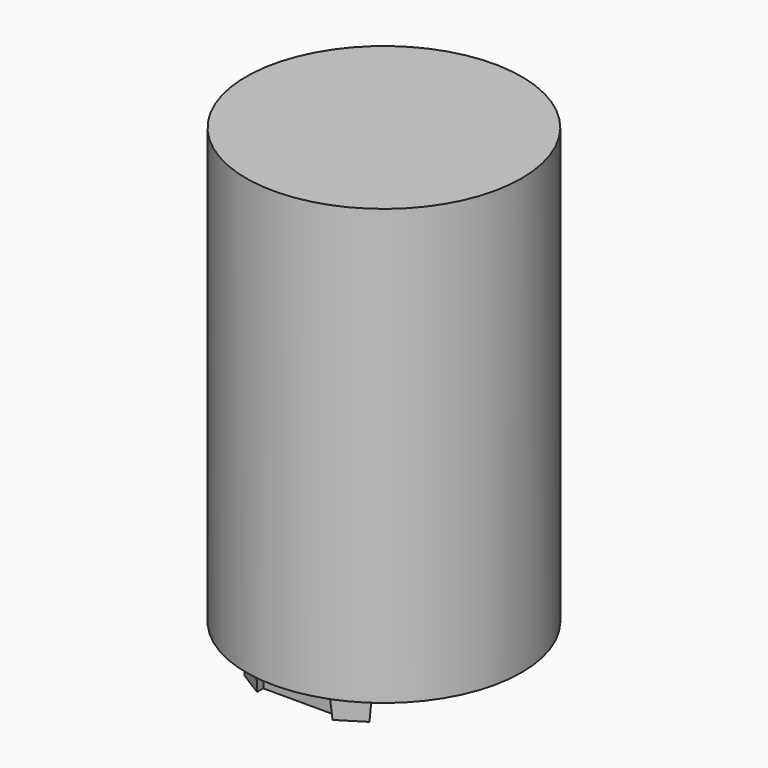
from build123d import *

# Parameters (mm, degrees)
F1_DEPTH = 2
F1_TAPER = 3
F0_R     = 9.5
F2_DEPTH = 30


with BuildPart() as f1:
    # F0 (on Top) → F1 (new body)
    with BuildSketch(Plane.XY):
        with BuildLine():
            Line((-2.5, -4.5), (-1.25, -4.5))
            Line((-1.25, -4.5), (-1.25, 8))
            ThreePointArc((-1.25, 8), (-1.6246096615, 8.4544378581), (-2.1421771094, 8.1734216623))
            Line((-2.1421771094, 8.1734216623), (-7.2625718321, -4.5))
            Line((-7.2625718321, -4.5), (-6.0125718321, -4.5))
            Line((-6.0125718321, -4.5), (-5.0025062675, -2))
            Line((-5.0025062675, -2), (-2.5, -2))
            Line((-2.5, -2), (-2.5, -4.5))
        make_face()
        Polygon((-2.5, -0.75), (-4.4974734852, -0.75), (-2.5, 4.1939203632), align=None, mode=Mode.SUBTRACT)
    extrude(amount=-F1_DEPTH, taper=F1_TAPER)


with BuildPart() as f1b:
    # F0 (on Top) → F1, piece 2 (new body)
    with BuildSketch(Plane.XY):
        with BuildLine():
            Line((1.25, 8.4544378581), (1.25, -4.5))
            ThreePointArc((1.25, -4.5), (5.075982109, -2.1148576985), (6.75, 2.0713944437))
            ThreePointArc((6.75, 2.0713944437), (5.1224940234, 6.2301220319), (1.25, 8.4544378581))
        make_face()
        with BuildLine():
            ThreePointArc((2.5, 6.7258275142), (4.6257418552, 4.8128070407), (5.4982695285, 2.0893678132))
            ThreePointArc((5.4982695285, 2.0893678132), (4.5914102703, -0.6620430511), (2.5, -2.6667022589))
            Line((2.5, -2.6667022589), (2.5, 6.7258275142))
        make_face(mode=Mode.SUBTRACT)
    extrude(amount=-F1_DEPTH, taper=F1_TAPER)


with BuildPart() as f1c:
    # F0 (on Top) → F1, piece 3 (new body)
    with BuildSketch(Plane.XY):
        Polygon((2.5, -6), (-2.5, -6), (-2.5, -5.375), (-4.5, -6.625), (-2.5, -7.875), (-2.5, -7.25), (2.5, -7.25), (2.5, -7.875), (4.5, -6.625), (2.5, -5.375), align=None)
    extrude(amount=-F1_DEPTH, taper=F1_TAPER)


with BuildPart() as f2:
    # F0 (on Top) → F2 (new body)
    with BuildSketch(Plane.XY):
        Circle(F0_R)
        Polygon((-2.5, -5.375), (-2.5, -6), (2.5, -6), (2.5, -5.375), (4.5, -6.625), (2.5, -7.875), (2.5, -7.25), (-2.5, -7.25), (-2.5, -7.875), (-4.5, -6.625), align=None, mode=Mode.SUBTRACT)
        with BuildLine():
            Line((-1.25, 8), (-1.25, -4.5))
            Line((-1.25, -4.5), (-2.5, -4.5))
            Line((-2.5, -4.5), (-2.5, -2))
            Line((-2.5, -2), (-5.0025062675, -2))
            Line((-5.0025062675, -2), (-6.0125718321, -4.5))
            Line((-6.0125718321, -4.5), (-7.2625718321, -4.5))
            Line((-7.2625718321, -4.5), (-2.1421771094, 8.1734216623))
            ThreePointArc((-2.1421771094, 8.1734216623), (-1.6246096615, 8.4544378581), (-1.25, 8))
        make_face(mode=Mode.SUBTRACT)
        with BuildLine():
            ThreePointArc((6.75, 2.0713944437), (5.075982109, -2.1148576985), (1.25, -4.5))
            Line((1.25, -4.5), (1.25, 8.4544378581))
            ThreePointArc((1.25, 8.4544378581), (5.1224940234, 6.2301220319), (6.75, 2.0713944437))
        make_face(mode=Mode.SUBTRACT)
        with BuildLine():
            Line((1.25, 8.4544378581), (1.25, -4.5))
            ThreePointArc((1.25, -4.5), (5.075982109, -2.1148576985), (6.75, 2.0713944437))
            ThreePointArc((6.75, 2.0713944437), (5.1224940234, 6.2301220319), (1.25, 8.4544378581))
        make_face()
        with BuildLine():
            ThreePointArc((2.5, 6.7258275142), (4.6257418552, 4.8128070407), (5.4982695285, 2.0893678132))
            ThreePointArc((5.4982695285, 2.0893678132), (4.5914102703, -0.6620430511), (2.5, -2.6667022589))
            Line((2.5, -2.6667022589), (2.5, 6.7258275142))
        make_face(mode=Mode.SUBTRACT)
        with BuildLine():
            Line((-2.5, -4.5), (-1.25, -4.5))
            Line((-1.25, -4.5), (-1.25, 8))
            ThreePointArc((-1.25, 8), (-1.6246096615, 8.4544378581), (-2.1421771094, 8.1734216623))
            Line((-2.1421771094, 8.1734216623), (-7.2625718321, -4.5))
            Line((-7.2625718321, -4.5), (-6.0125718321, -4.5))
            Line((-6.0125718321, -4.5), (-5.0025062675, -2))
            Line((-5.0025062675, -2), (-2.5, -2))
            Line((-2.5, -2), (-2.5, -4.5))
        make_face()
        Polygon((-2.5, -0.75), (-4.4974734852, -0.75), (-2.5, 4.1939203632), align=None, mode=Mode.SUBTRACT)
        with BuildLine():
            ThreePointArc((2.5, -2.6667022589), (4.5914102703, -0.6620430511), (5.4982695285, 2.0893678132))
            ThreePointArc((5.4982695285, 2.0893678132), (4.6257418552, 4.8128070407), (2.5, 6.7258275142))
            Line((2.5, 6.7258275142), (2.5, -2.6667022589))
        make_face()
        Polygon((2.5, -6), (-2.5, -6), (-2.5, -5.375), (-4.5, -6.625), (-2.5, -7.875), (-2.5, -7.25), (2.5, -7.25), (2.5, -7.875), (4.5, -6.625), (2.5, -5.375), align=None)
        Polygon((-2.5, 4.1939203632), (-4.4974734852, -0.75), (-2.5, -0.75), align=None)
    extrude(amount=F2_DEPTH)


solid = Compound([f1.part, f1b.part, f1c.part, f2.part])
